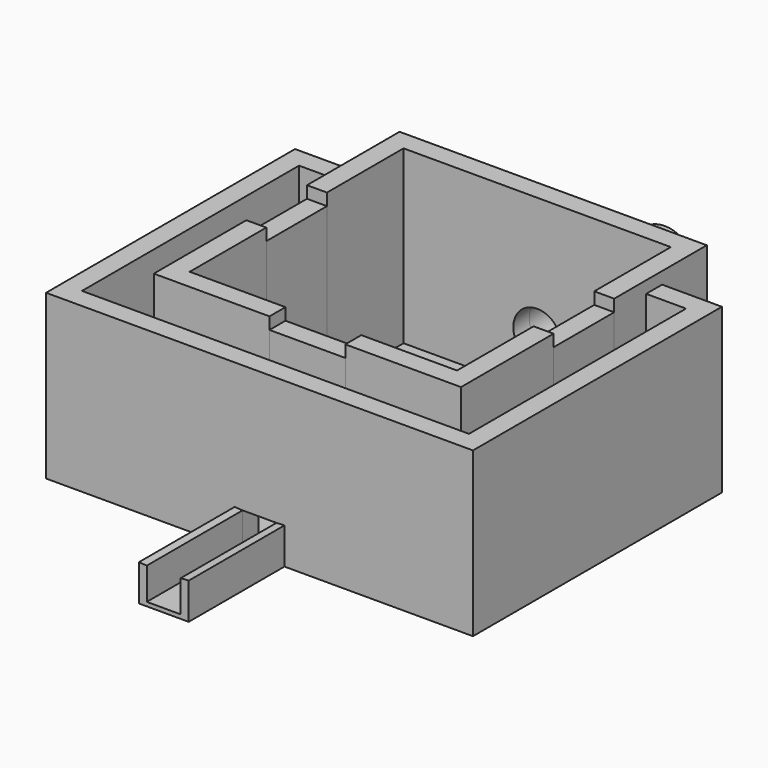
from build123d import *

# Parameters (mm, degrees)
F1_DEPTH  = 44
F0_W      = 5
F0_H      = 19
F2_DEPTH  = 41
F0_W_2    = 19
F0_H_2    = 5
F0_W_3    = 8.5
F3_DEPTH  = 41
F4_DEPTH  = 1
F5_R      = 8
F5_R_2    = 6
F6_DEPTH  = 35
F7_DEPTH  = 25
F8_W      = 8.5
F8_H      = 1
F8_W_2    = 2
F9_DEPTH  = 30
F8_H_2    = 8
F10_DEPTH = 25


with BuildPart() as f1:
    # F0 (on Top) → F1 (new body)
    with BuildSketch(Plane.XY):
        Polygon((-33.5, 33.5), (33.5, 33.5), (33.5, 9.5), (38.5, 9.5), (38.5, 19.5), (38.5, 24.5), (38.5, 38.5), (6, 38.5), (-6, 38.5), (-38.5, 38.5), (-38.5, 24.5), (-38.5, 19.5), (-38.5, 9.5), (-33.5, 9.5), align=None)
    extrude(amount=F1_DEPTH)

    # F0 (on Top) → F3 (join)
    with BuildSketch(Plane.XY):
        Polygon((-48.5, 19.5), (-38.5, 19.5), (-38.5, 24.5), (-53.5, 24.5), (-53.5, 19.5), (-53.5, -53.5), (-4.25, -53.5), (-4.25, -48.5), (-48.5, -48.5), align=None)
        Polygon((38.5, 24.5), (38.5, 19.5), (48.5, 19.5), (48.5, -48.5), (4.25, -48.5), (4.25, -53.5), (53.5, -53.5), (53.5, 19.5), (53.5, 24.5), align=None)
        with Locations((0, -51)):
            Rectangle(F0_W_3, F0_H_2)
    extrude(amount=F3_DEPTH)

    # F5 (on face) → F6 (join)
    with BuildSketch(Plane(origin=(0, 38.5, 0), x_dir=(-1, 0, 0), z_dir=(0, 1, 0))):
        with Locations((0, 13.5)):
            Circle(F5_R)
        with Locations((0, 13.5)):
            Circle(F5_R_2, mode=Mode.SUBTRACT)
    extrude(amount=F6_DEPTH)

    # F7 (cut): a face of the model
    f7_faces = [f1.faces().sort_by_distance(p)[0] for p in [
        (0, 38.5, 13.5),
    ]]
    extrude(f7_faces, amount=-F7_DEPTH, mode=Mode.SUBTRACT)

    # F8 (on face) → F9 (join)
    with BuildSketch(Plane.XZ.offset(53.5)):
        with Locations((0, 0.5)):
            Rectangle(F8_W, F8_H)
        Polygon((4.25, 9), (4.25, 1), (6.25, 1), (6.25, 9.1), align=None)
        Polygon((-6.25, 1), (-4.25, 1), (-4.25, 9), (-6.25, 9.1), align=None)
        with Locations((5.25, 0.5)):
            Rectangle(F8_W_2, F8_H)
        with Locations((-5.25, 0.5)):
            Rectangle(F8_W_2, F8_H)
    extrude(amount=F9_DEPTH)

    # F8 (on face) → F10 (cut)
    with BuildSketch(Plane.XZ.offset(53.5)):
        with Locations((0, 5)):
            Rectangle(F8_W, F8_H_2)
    extrude(amount=-F10_DEPTH, mode=Mode.SUBTRACT)


with BuildPart() as f1b:
    # F0 (on Top) → F1, piece 2 (new body)
    with BuildSketch(Plane.XY):
        Polygon((-33.5, -33.5), (-33.5, -9.5), (-38.5, -9.5), (-38.5, -38.5), (-9.5, -38.5), (-9.5, -33.5), align=None)
    extrude(amount=F1_DEPTH)


with BuildPart() as f1c:
    # F0 (on Top) → F1, piece 3 (new body)
    with BuildSketch(Plane.XY):
        Polygon((38.5, -9.5), (33.5, -9.5), (33.5, -33.5), (9.5, -33.5), (9.5, -38.5), (38.5, -38.5), align=None)
    extrude(amount=F1_DEPTH)


with BuildPart() as f2:
    # F0 (on Top) → F2 (new body)
    with BuildSketch(Plane.XY):
        with Locations((-36, 0)):
            Rectangle(F0_W, F0_H)
    extrude(amount=F2_DEPTH)


with BuildPart() as f2b:
    # F0 (on Top) → F2, piece 2 (new body)
    with BuildSketch(Plane.XY):
        with Locations((36, 0)):
            Rectangle(F0_W, F0_H)
    extrude(amount=F2_DEPTH)


with BuildPart() as f2c:
    # F0 (on Top) → F2, piece 3 (new body)
    with BuildSketch(Plane.XY):
        with Locations((0, -36)):
            Rectangle(F0_W_2, F0_H_2)
    extrude(amount=F2_DEPTH)


with BuildPart() as f4:
    # F0 (on Top) → F4 (new body)
    with BuildSketch(Plane.XY):
        Polygon((33.5, 9.5), (33.5, 33.5), (-33.5, 33.5), (-33.5, 9.5), (-33.5, -9.5), (-33.5, -33.5), (-9.5, -33.5), (9.5, -33.5), (33.5, -33.5), (33.5, -9.5), align=None)
    extrude(amount=F4_DEPTH)


with BuildPart() as f4b:
    # F0 (on Top) → F4, piece 2 (new body)
    with BuildSketch(Plane.XY):
        Polygon((38.5, 19.5), (38.5, 9.5), (38.5, -9.5), (38.5, -38.5), (9.5, -38.5), (-9.5, -38.5), (-38.5, -38.5), (-38.5, -9.5), (-38.5, 9.5), (-38.5, 19.5), (-48.5, 19.5), (-48.5, -48.5), (-4.25, -48.5), (4.25, -48.5), (48.5, -48.5), (48.5, 19.5), align=None)
    extrude(amount=F4_DEPTH)


solid = Compound([f1.part, f1b.part, f1c.part, f2.part, f2b.part, f2c.part, f4.part, f4b.part])
